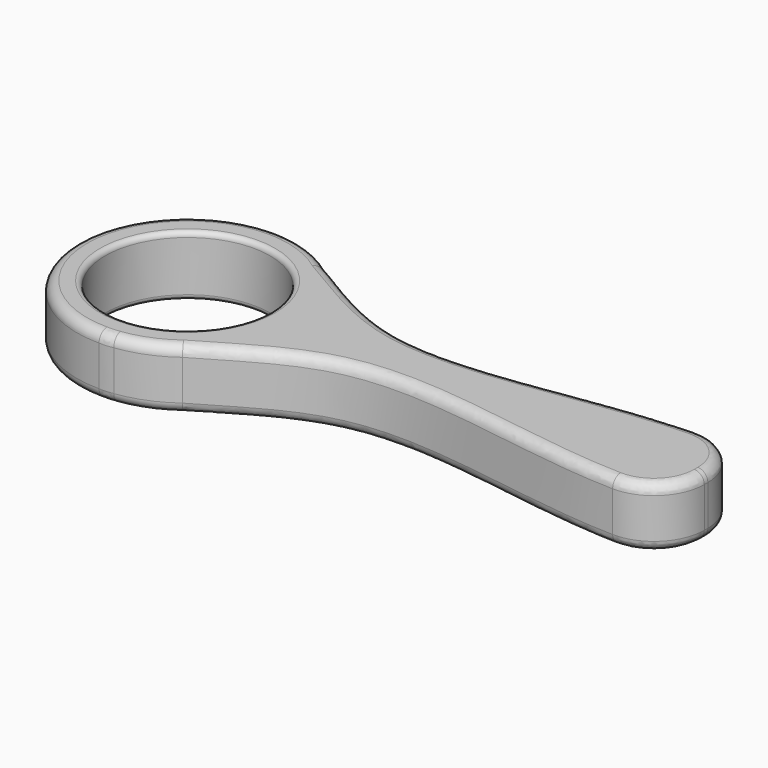
from build123d import *

# Parameters (mm, degrees)
F0_R     = 8.2
F1_DEPTH = 6
F2_R     = 5
F3_R     = 1
F4_R     = 0.5
F5_R     = 0.5


# Not quite as in the source:
# - a feature names something its author has since deleted; it is built from what else it names


with BuildPart() as f1:
    # F0 (on Top) → F1 (new body)
    with BuildSketch(Plane.XY):
        with BuildLine():
            ThreePointArc((1.3913431653, 10.9116526794), (0.6970726384, 10.9778909512), (0, 11))
            ThreePointArc((0, 11), (-11, 0), (0, -11))
            ThreePointArc((0, -11), (0.6970726384, -10.9778909512), (1.3913431653, -10.9116526794))
            add(Edge.make_bspline(
                [(1.3913431653, -10.9116526794), (3.0665996188, -10.6457430697), (4.7711138609, -9.836379326), (6.5606813815, -8.8293521739)],
                knots=[0.0382275962, 0.0382275962, 0.0382275962, 0.0382275962, 0.1757603333, 0.1757603333, 0.1757603333, 0.1757603333], degree=3))
            ThreePointArc((6.5606813815, -8.8293521739), (9.8277030683, -4.9412804415), (11, 0))
            ThreePointArc((11, 0), (9.8277030683, 4.9412804415), (6.5606813815, 8.8293521739))
            add(Edge.make_bspline(
                [(1.3913431653, 10.9116526794), (3.0665996188, 10.6457430697), (4.7711138609, 9.836379326), (6.5606813815, 8.8293521739)],
                knots=[0.0382275962, 0.0382275962, 0.0382275962, 0.0382275962, 0.1757603333, 0.1757603333, 0.1757603333, 0.1757603333], degree=3))
        make_face()
        Circle(F0_R, mode=Mode.SUBTRACT)
        with BuildLine():
            add(Edge.make_bspline(
                [(0, 11), (0.4623194333, 11.0174872499), (0.9257011045, 10.9855629744), (1.3913431653, 10.9116526794)],
                knots=[0, 0, 0, 0, 0.0382275962, 0.0382275962, 0.0382275962, 0.0382275962], degree=3))
            ThreePointArc((0, 11), (0.6970726384, 10.9778909512), (1.3913431653, 10.9116526794))
        make_face()
        with BuildLine():
            ThreePointArc((1.3913431653, -10.9116526794), (0.6970726384, -10.9778909512), (0, -11))
            add(Edge.make_bspline(
                [(0, -11), (0.4623194333, -11.0174872499), (0.9257011045, -10.9855629744), (1.3913431653, -10.9116526794)],
                knots=[0, 0, 0, 0, 0.0382275962, 0.0382275962, 0.0382275962, 0.0382275962], degree=3))
        make_face()
        with BuildLine():
            ThreePointArc((6.5606813815, 8.8293521739), (4.1100690319, 10.2033000815), (1.3913431653, 10.9116526794))
            add(Edge.make_bspline(
                [(1.3913431653, 10.9116526794), (3.0665996188, 10.6457430697), (4.7711138609, 9.836379326), (6.5606813815, 8.8293521739)],
                knots=[0.0382275962, 0.0382275962, 0.0382275962, 0.0382275962, 0.1757603333, 0.1757603333, 0.1757603333, 0.1757603333], degree=3))
        make_face()
        with BuildLine():
            add(Edge.make_bspline(
                [(1.3913431653, -10.9116526794), (3.0665996188, -10.6457430697), (4.7711138609, -9.836379326), (6.5606813815, -8.8293521739)],
                knots=[0.0382275962, 0.0382275962, 0.0382275962, 0.0382275962, 0.1757603333, 0.1757603333, 0.1757603333, 0.1757603333], degree=3))
            ThreePointArc((1.3913431653, -10.9116526794), (4.1100690319, -10.2033000815), (6.5606813815, -8.8293521739))
        make_face()
        with BuildLine():
            add(Edge.make_bspline(
                [(6.5606813815, 8.8293521739), (9.8676903183, 6.9684289321), (21.5345916566, -1.2558052526), (39.9595495481, 6.3712443804), (51.5451952815, 5)],
                knots=[0.1757603333, 0.1757603333, 0.1757603333, 0.1757603333, 0.4299122364, 1, 1, 1, 1], degree=3))
            ThreePointArc((6.5606813815, 8.8293521739), (9.8277030683, 4.9412804415), (11, 0))
            ThreePointArc((11, 0), (9.8277030683, -4.9412804415), (6.5606813815, -8.8293521739))
            add(Edge.make_bspline(
                [(6.5606813815, -8.8293521739), (9.8676903183, -6.9684289321), (21.5345916566, 1.2558052526), (39.9595495481, -6.3712443804), (51.5451952815, -5)],
                knots=[0.1757603333, 0.1757603333, 0.1757603333, 0.1757603333, 0.4299122364, 1, 1, 1, 1], degree=3))
            Line((51.5451952815, -5), (51.5451952815, 5))
        make_face()
    extrude(amount=F1_DEPTH)

    # F2
    f2_edges = [f1.edges().sort_by_distance(p)[0] for p in [
        (51.545195, -5, 3),
        (51.545195, 5, 3),
    ]]
    fillet(f2_edges, radius=F2_R)

    # F3
    f3_edges = [f1.edges().sort_by_distance(p)[0] for p in [
        (-11, 0, 6),
        (-11, 0, 0),
        (23.906379, -2.817553, 0),
        (23.906379, -2.817553, 6),
        (50.041708, -3.795751, 0),
        (4.110069, -10.2033, 0),
        (51.545195, 0, 0),
        (0.694426, -10.9901, 0),
        (50.041708, 3.795751, 0),
        (23.906379, 2.817553, 0),
        (0.694426, 10.9901, 0),
        (4.110069, 10.2033, 0),
        (50.041708, -3.795751, 6),
        (4.110069, -10.2033, 6),
        (51.545195, 0, 6),
        (0.694426, -10.9901, 6),
        (50.041708, 3.795751, 6),
        (23.906379, 2.817553, 6),
        (0.694426, 10.9901, 6),
        (4.110069, 10.2033, 6),
    ]]
    fillet(f3_edges, radius=F3_R)

    # F4
    f4_edges = [f1.edges().sort_by_distance(p)[0] for p in [
        (-8.2, 0, 0),
    ]]
    fillet(f4_edges, radius=F4_R)

    # F5
    f5_edges = [f1.edges().sort_by_distance(p)[0] for p in [
        (-8.2, 0, 6),
    ]]
    fillet(f5_edges, radius=F5_R)


solid = f1.part
